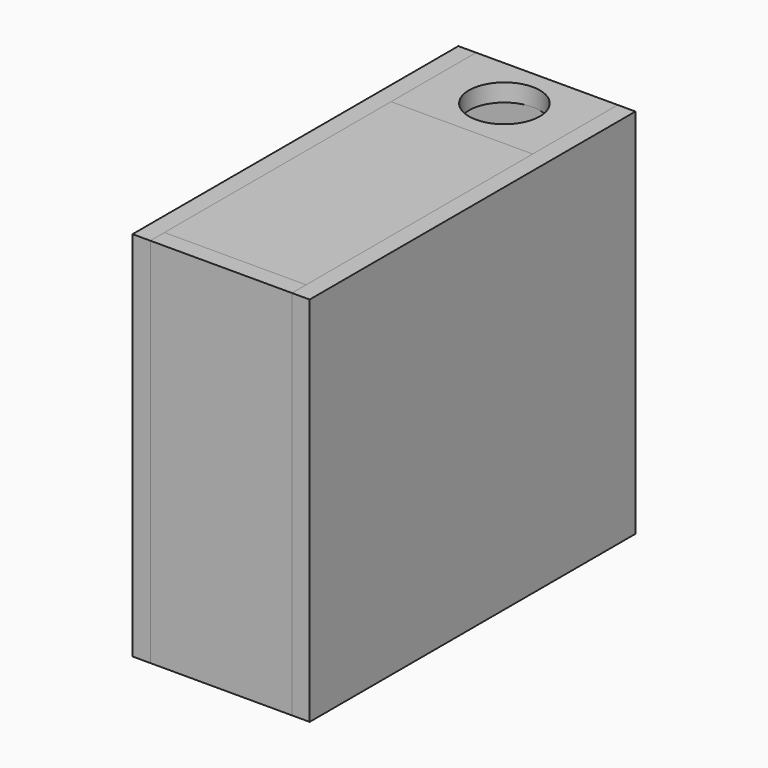
from build123d import *

# Parameters (mm, degrees)
F0_W      = 101.6
F0_H      = 127
F1_DEPTH  = 50.8
F2_W      = 6.35
F2_H      = 95.25
F3_DEPTH  = 50.8
F4_W      = 146.05
F4_H      = 133.35
F5_DEPTH  = 6.35
F9_R      = 12.7
F10_DEPTH = 6.35


# Not quite as in the source:
# - a feature names something its author has since deleted; it is built from what else it names


with BuildPart() as f1:
    # F0 (on Right) → F1 (new body)
    with BuildSketch(Plane.YZ):
        with Locations((0, 63.5)):
            Rectangle(F0_W, F0_H)
    extrude(amount=-F1_DEPTH)


with BuildPart() as f3:
    # F2 (on face) → F3 (new body, through all)
    with BuildSketch(Plane(origin=(-50.8, 0, 0), x_dir=(0, -1, 0), z_dir=(-1, 0, 0))):
        Polygon((50.8, 127), (50.8, 0), (-82.55, 0), (-82.55, 120.65), (-57.15, 120.65), (-50.8, 120.65), (-50.8, 127), (-82.55, 127), (-88.9, 127), (-88.9, 0), (-88.9, -6.35), (57.15, -6.35), (57.15, 127), align=None)
        with Locations((-53.975, 73.025)):
            Rectangle(F2_W, F2_H)
    extrude(amount=-F3_DEPTH)

    # F9 (on face) → F10 (cut)
    with BuildSketch(Plane.XY.offset(127)):
        with Locations((-25.4, 69.85)):
            Circle(F9_R)
    extrude(amount=-F10_DEPTH, mode=Mode.SUBTRACT)


with BuildPart() as f5:
    # F4 (on face) → F5 (new body)
    with BuildSketch(Plane(origin=(-50.8, 0, 0), x_dir=(0, -1, 0), z_dir=(-1, 0, 0))):
        with Locations((-15.875, 60.325)):
            Rectangle(F4_W, F4_H)
    extrude(amount=F5_DEPTH)


with BuildPart() as f8_1:
    # F8: instance of F5
    add(f5.part.mirror(Plane(origin=(-25.4, 15.875, 60.325), x_dir=(0, -1, 0), z_dir=(1, 0, 0))))


solid = Compound([f1.part, f3.part, f5.part, f8_1.part])
